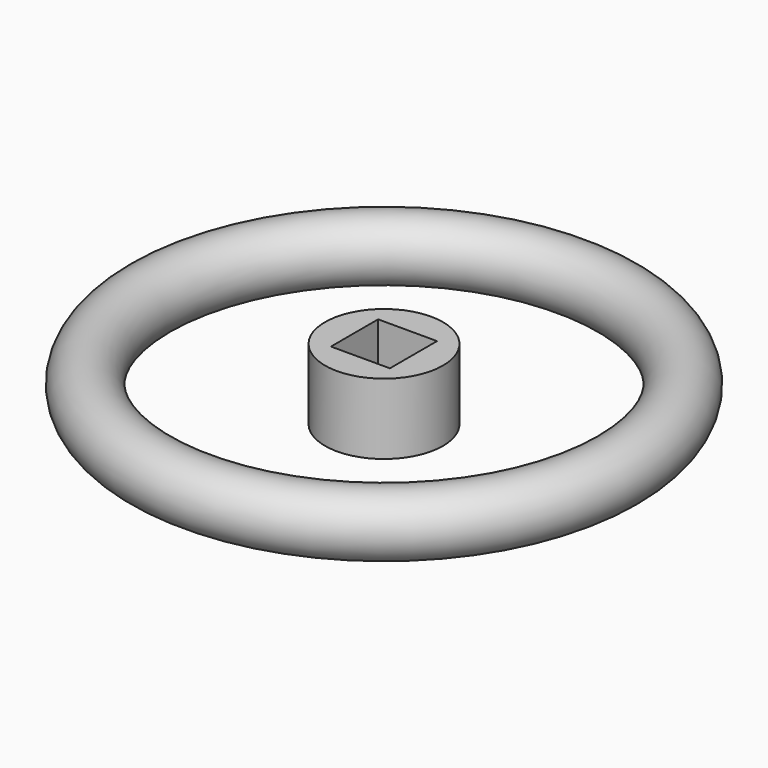
from build123d import *

# Parameters (mm, degrees)
F0_R     = 13
F2_R     = 25
F2_W     = 25
F2_H     = 25
F3_DEPTH = 15


# Not quite as in the source:
# - a feature of the source that left no trace in its solid (it failed there, or was rolled back) is left out
# - the program builds the solid bodies; features that only make, move or delete a surface that nothing else refers to are left out


with BuildPart() as f1:
    # F0 (on Front) → F1 (revolve)
    with BuildSketch(Plane.XZ):
        with Locations((-99, 0)):
            Circle(F0_R)
    revolve(axis=Axis((0, 0, -6.8144798279), (0, 0, -1)))


with BuildPart() as f3:
    # F2 (on Top) → F3 (new body, symmetric)
    with BuildSketch(Plane.XY):
        Circle(F2_R)
        Rectangle(F2_W, F2_H, mode=Mode.SUBTRACT)
    extrude(amount=F3_DEPTH, both=True)


solid = Compound([f1.part, f3.part])
